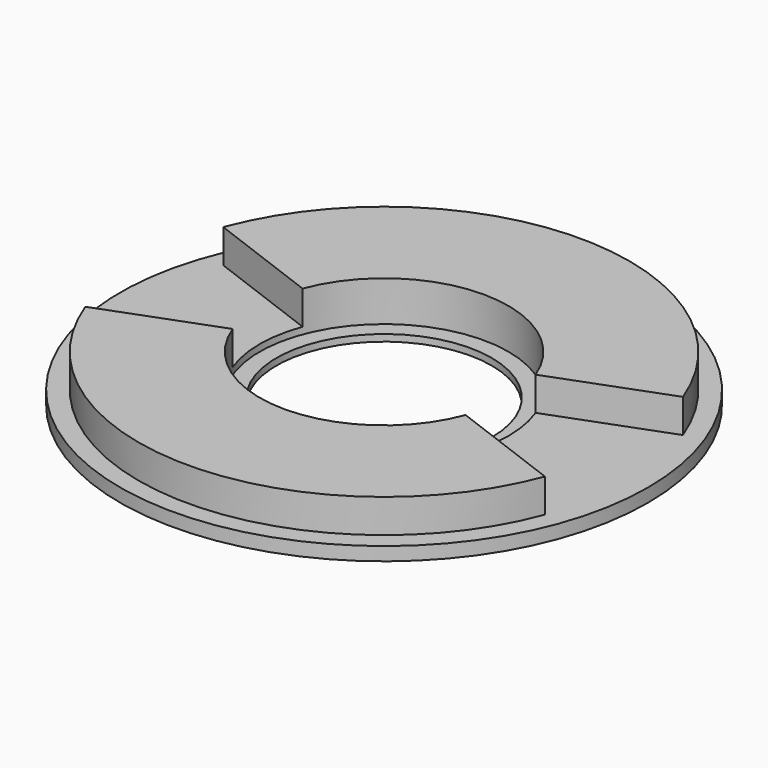
from build123d import *

# Parameters (mm, degrees)
F0_R     = 36.5
F0_R_2   = 31.5
F1_DEPTH = 7
F0_R_3   = 39.25
F2_DEPTH = 2
F3_R     = 18.5
F3_R_2   = 16
F4_DEPTH = 6
F5_DEPTH = 25
F7_DEPTH = 5


with BuildPart() as f1:
    # F0 (on Top) → F1 (new body)
    with BuildSketch(Plane.XY):
        Circle(F0_R)
        Circle(F0_R_2, mode=Mode.SUBTRACT)
        Circle(F0_R_2)
    extrude(amount=F1_DEPTH)

    # F0 (on Top) → F2 (join)
    with BuildSketch(Plane.XY):
        Circle(F0_R_3)
        Circle(F0_R, mode=Mode.SUBTRACT)
        Circle(F0_R)
        Circle(F0_R_2, mode=Mode.SUBTRACT)
    extrude(amount=F2_DEPTH)

    # F3 (on face) → F4 (cut)
    with BuildSketch(Plane.XY.offset(7)):
        Circle(F3_R)
        Circle(F3_R_2, mode=Mode.SUBTRACT)
        Circle(F3_R_2)
    extrude(amount=-F4_DEPTH, mode=Mode.SUBTRACT)

    # F3 (on face) → F5 (cut)
    with BuildSketch(Plane.XY.offset(7)):
        Circle(F3_R_2)
    extrude(amount=-F5_DEPTH, mode=Mode.SUBTRACT)

    # F6 (on face) → F7 (cut)
    with BuildSketch(Plane.XY.offset(7)):
        Polygon((17.3205080757, -6.5), (40, -6.5), (40, 6.5), (17.3205080757, 6.5), (-17.3205080757, 6.5), (-40, 6.5), (-40, -6.5), (-17.3205080757, -6.5), align=None)
        with BuildLine():
            Line((-35.9165699921, 6.5), (-17.3205080757, 6.5))
            Line((-17.3205080757, 6.5), (-34.1728943115, 12.8243243243))
            ThreePointArc((-34.1728943115, 12.8243243243), (-35.1871073141, 9.7014163331), (-35.9165699921, 6.5))
        make_face()
        with BuildLine():
            Line((-34.1728943115, -12.8243243243), (-17.3205080757, -6.5))
            Line((-17.3205080757, -6.5), (-35.9165699921, -6.5))
            ThreePointArc((-35.9165699921, -6.5), (-35.1871073141, -9.7014163331), (-34.1728943115, -12.8243243243))
        make_face()
        with BuildLine():
            Line((35.9165699921, -6.5), (17.3205080757, -6.5))
            Line((17.3205080757, -6.5), (34.1728943115, -12.8243243243))
            ThreePointArc((34.1728943115, -12.8243243243), (35.1871073141, -9.7014163331), (35.9165699921, -6.5))
        make_face()
        with BuildLine():
            Line((34.1728943115, 12.8243243243), (17.3205080757, 6.5))
            Line((17.3205080757, 6.5), (35.9165699921, 6.5))
            ThreePointArc((35.9165699921, 6.5), (35.1871073141, 9.7014163331), (34.1728943115, 12.8243243243))
        make_face()
    extrude(amount=-F7_DEPTH, mode=Mode.SUBTRACT)


solid = f1.part
